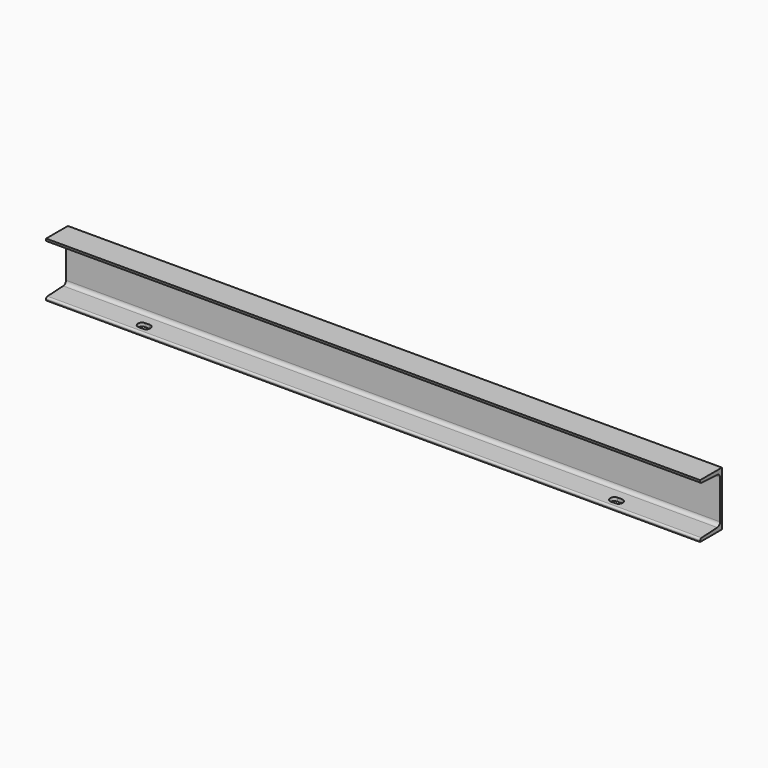
from build123d import *

# Parameters (mm, degrees)
F1_DEPTH = 1800
F3_DEPTH = 9.9223883311


# Not quite as in the source:
# - a pattern or mirror of a feature is missing from the dataset's text; its kind, count and spacing are read off the source's solid


with BuildPart() as f1:
    # F0 (on Right) → F1 (new body)
    with BuildSketch(Plane.YZ):
        with BuildLine():
            Line((185.4237287785, 0), (110.4237287785, 0))
            Line((110.4237287785, 0), (110.4237287785, -3.2898854433))
            ThreePointArc((110.4237287785, -3.2898854433), (111.7968569235, -6.7316583218), (115.1620489973, -8.2830331171))
            Line((115.1620489973, -8.2830331171), (169.447088341, -11.1279914774))
            ThreePointArc((169.447088341, -11.1279914774), (176.1774724886, -14.230741068), (178.9237287785, -21.1142868249))
            Line((178.9237287785, -21.1142868249), (178.9237287785, -128.8857131751))
            ThreePointArc((178.9237287785, -128.8857131751), (176.1774724886, -135.769258932), (169.447088341, -138.8720085226))
            Line((169.447088341, -138.8720085226), (115.1620489973, -141.7169668829))
            ThreePointArc((115.1620489973, -141.7169668829), (111.7968569235, -143.2683416782), (110.4237287785, -146.7101145567))
            Line((110.4237287785, -146.7101145567), (110.4237287785, -150))
            Line((110.4237287785, -150), (185.4237287785, -150))
            Line((185.4237287785, -150), (185.4237287785, 0))
        make_face()
    extrude(amount=F1_DEPTH)

    # F2 (on face) → F3 (cut, through all)
    with BuildSketch(Plane(origin=(0, 0, -150), x_dir=(1, 0, 0), z_dir=(0, 0, -1))):
        with BuildLine():
            ThreePointArc((243.5, -124.4237287785), (232.5, -135.4237287785), (243.5, -146.4237287785))
            Line((243.5, -146.4237287785), (256.5, -146.4237287785))
            ThreePointArc((256.5, -146.4237287785), (267.5, -135.4237287785), (256.5, -124.4237287785))
            Line((256.5, -124.4237287785), (243.5, -124.4237287785))
        make_face()
    f3 = extrude(amount=-F3_DEPTH, mode=Mode.SUBTRACT)

    # F3_copies: F3 across plane
    add(f3.mirror(Plane(origin=(900, 0, 0), x_dir=(0, 0, 1), z_dir=(1, 0, 0))), mode=Mode.SUBTRACT)


solid = f1.part
